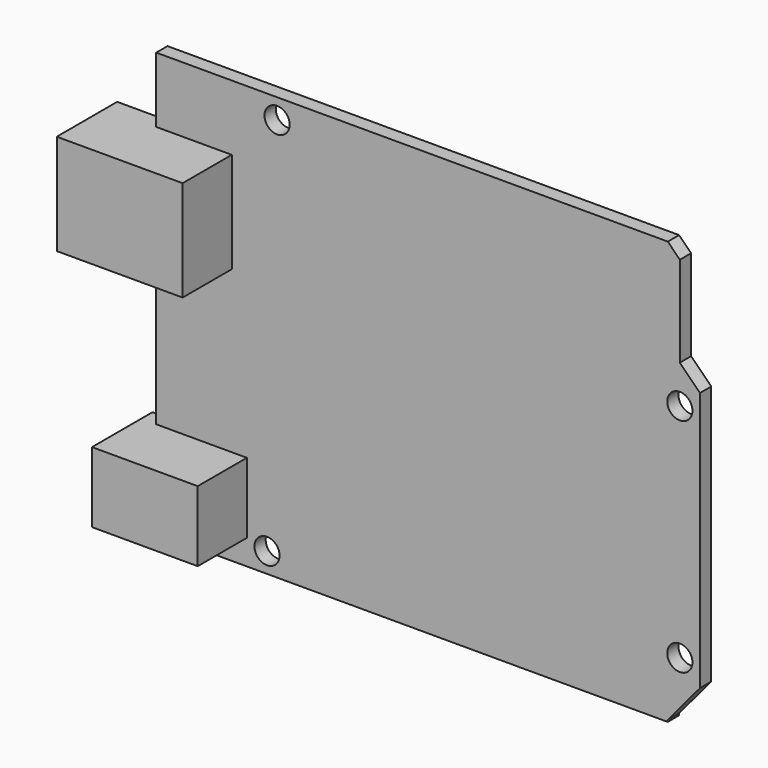
from build123d import *

# Parameters (mm, degrees)
F0_R     = 1.5875
F1_DEPTH = 1.778
F0_W     = 6.35
F0_H     = 12.7
F0_W_2   = 9.525
F2_DEPTH = 9.525
F0_W_3   = 11.43
F0_H_2   = 8.89
F0_W_4   = 1.905


# Not quite as in the source:
# - ends of sketch curves that miss each other by under 0.0002 mm in the source are joined


with BuildPart() as f1:
    # F0 (on Front) → F1 (new body)
    with BuildSketch(Plane.XZ):
        Polygon((15.6624242663, 58.1459343719), (-48.8660596311, 58.1459343719), (-48.8660596311, 49.8909343719), (-39.3410596311, 49.8909343719), (-39.3410596311, 37.1909343719), (-48.8660596311, 37.1909343719), (-48.8660596311, 16.8709343719), (-37.4360596311, 16.8709343719), (-37.4360596311, 7.9809343719), (-48.8660596311, 7.9809343719), (-48.8660596311, 4.8059343719), (15.6499403689, 4.8059343719), (15.6499403689, 5.0407722592), (19.7139403689, 9.8859343719), (19.7139403689, 42.6519343719), (17.1739701182, 45.1919343719), (17.1739701182, 56.6219343719), align=None)
        with Locations((-34.8960596311, 7.3459343719)):
            Circle(F0_R, mode=Mode.SUBTRACT)
        with Locations((17.1739403689, 12.4259343719)):
            Circle(F0_R, mode=Mode.SUBTRACT)
        with Locations((-33.6260596311, 55.6059343719)):
            Circle(F0_R, mode=Mode.SUBTRACT)
        with Locations((17.1739403689, 40.3659343719)):
            Circle(F0_R, mode=Mode.SUBTRACT)
    extrude(amount=F1_DEPTH)


with BuildPart() as f2:
    # F0 (on Front) → F2 (new body)
    with BuildSketch(Plane.XZ):
        with Locations((-52.0410596311, 43.5409343719)):
            Rectangle(F0_W, F0_H)
        with Locations((-44.1035596311, 43.5409343719)):
            Rectangle(F0_W_2, F0_H)
    extrude(amount=F2_DEPTH)


with BuildPart() as f2b:
    # F0 (on Front) → F2, piece 2 (new body)
    with BuildSketch(Plane.XZ):
        with Locations((-43.1510596311, 12.4259343719)):
            Rectangle(F0_W_3, F0_H_2)
        with Locations((-49.8185596311, 12.4259343719)):
            Rectangle(F0_W_4, F0_H_2)
    extrude(amount=F2_DEPTH)


solid = Compound([f1.part, f2.part, f2b.part])
